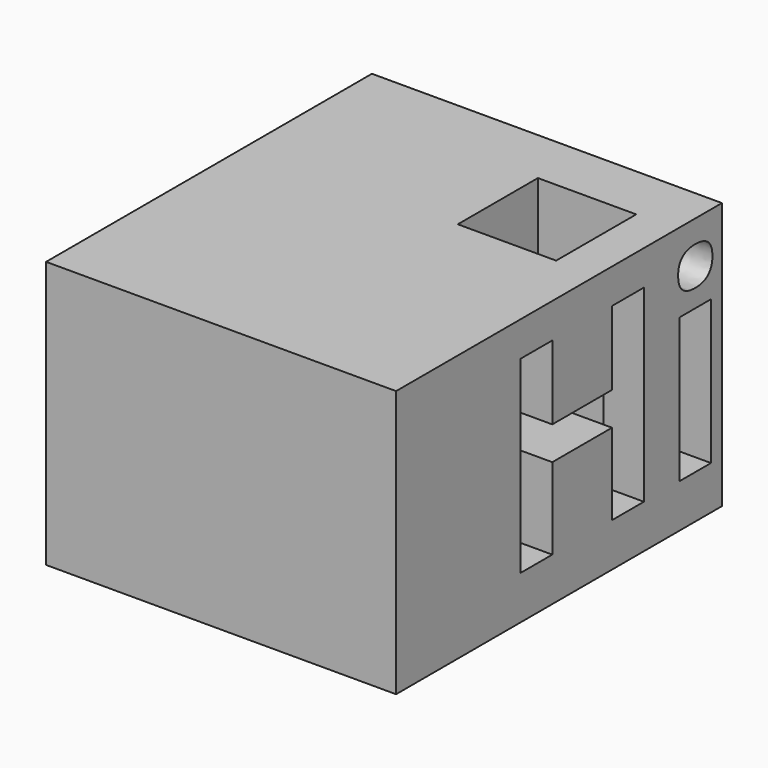
from build123d import *

# Parameters (mm, degrees)
F0_W         = 66.62543118
F0_H         = 77.5313749909
F1_DEPTH     = 50.8
F2_W         = 18.7210184522
F2_H         = 19.059448503
F3_DEPTH     = 50.8
F4_TEXT_SIZE = 50.2785822997
F5_DEPTH     = 25.4


# Not quite as in the source:
# - Text() gives the source's letters only with a copy of the font that has no kerning and outlines rounded to 1/6400 em; it was checked with that copy


with BuildPart() as f1:
    # F0 (on Top) → F1 (new body)
    with BuildSketch(Plane.XY):
        Rectangle(F0_W, F0_H)
    extrude(amount=F1_DEPTH)

    # F2 (on Top) → F3 (cut, through all)
    with BuildSketch(Plane.XY):
        with Locations((16.2864585873, 18.4299093671)):
            Rectangle(F2_W, F2_H)
    extrude(amount=F3_DEPTH, mode=Mode.SUBTRACT)

    # F4 (on face) → F5 (cut)
    with BuildSketch(Plane.YZ.offset(33.31271559)):
        with Locations((-13.7272300199, 8.2905627787)):
            Text('Hi', F4_TEXT_SIZE, font='Open Sans', font_style=FontStyle.BOLD, text_align=(TextAlign.LEFT, TextAlign.BOTTOM))
    extrude(amount=-F5_DEPTH, mode=Mode.SUBTRACT)


solid = f1.part
